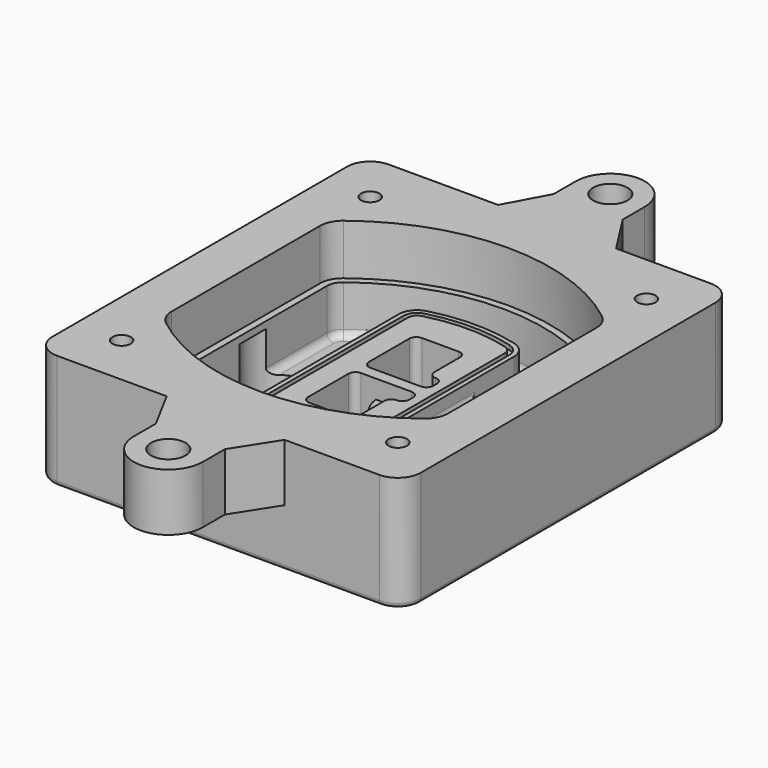
from build123d import *

# Parameters (mm, degrees)
F0_R      = 4
F1_DEPTH  = 25
F2_DEPTH  = 3
F3_DEPTH  = 18
F5_DEPTH  = 21
F6_DEPTH  = 2
F8_DEPTH  = 20
F9_DEPTH  = 16
F10_DEPTH = 25
F7_R      = 6
F7_R_2    = 4
F11_DEPTH = 6
F13_DEPTH = 9
F14_R     = 3
F15_R     = 2
F16_R     = 4
F17_DEPTH = 25
F18_DEPTH = 25
F19_DEPTH = 25
F16_R_2   = 7.5
F20_DEPTH = 25


# Not quite as in the source:
# - a feature names something its author has since deleted; it is built from what else it names


with BuildPart() as f1:
    # F0 (on Top) → F1 (new body)
    with BuildSketch(Plane.XY):
        with BuildLine():
            ThreePointArc((-80, -80), (-77.0710678119, -87.0710678119), (-70, -90))
            Line((-70, -90), (70, -90))
            ThreePointArc((70, -90), (77.0710678119, -87.0710678119), (80, -80))
            Line((80, -80), (80, 80))
            ThreePointArc((80, 80), (77.0710678119, 87.0710678119), (70, 90))
            Line((70, 90), (-70, 90))
            ThreePointArc((-70, 90), (-77.0710678119, 87.0710678119), (-80, 80))
            Line((-80, 80), (-80, -80))
        make_face()
        with Locations((-60, -67.5)):
            Circle(F0_R, mode=Mode.SUBTRACT)
        with Locations((60, -67.5)):
            Circle(F0_R, mode=Mode.SUBTRACT)
        with Locations((-60, 67.5)):
            Circle(F0_R, mode=Mode.SUBTRACT)
        with BuildLine():
            ThreePointArc((-64, 40.2934422872), (-62.5820384798, 46.4328484224), (-58.6153846154, 51.3286200352))
            ThreePointArc((-58.6153846154, 51.3286200352), (0, 71.5), (58.6153846154, 51.3286200352))
            ThreePointArc((58.6153846154, 51.3286200352), (62.5820384798, 46.4328484224), (64, 40.2934422872))
            Line((64, 40.2934422872), (64, -40.2934422872))
            ThreePointArc((64, -40.2934422872), (62.5820384798, -46.4328484224), (58.6153846154, -51.3286200352))
            ThreePointArc((58.6153846154, -51.3286200352), (0, -71.5), (-58.6153846154, -51.3286200352))
            ThreePointArc((-58.6153846154, -51.3286200352), (-62.5820384798, -46.4328484224), (-64, -40.2934422872))
            Line((-64, -40.2934422872), (-64, 40.2934422872))
        make_face(mode=Mode.SUBTRACT)
        with Locations((60, 67.5)):
            Circle(F0_R, mode=Mode.SUBTRACT)
        with BuildLine():
            ThreePointArc((58.6153846154, 51.3286200352), (0, 71.5), (-58.6153846154, 51.3286200352))
            ThreePointArc((-58.6153846154, 51.3286200352), (-62.5820384798, 46.4328484224), (-64, 40.2934422872))
            Line((-64, 40.2934422872), (-64, -40.2934422872))
            ThreePointArc((-64, -40.2934422872), (-62.5820384798, -46.4328484224), (-58.6153846154, -51.3286200352))
            ThreePointArc((-58.6153846154, -51.3286200352), (0, -71.5), (58.6153846154, -51.3286200352))
            ThreePointArc((58.6153846154, -51.3286200352), (62.5820384798, -46.4328484224), (64, -40.2934422872))
            Line((64, -40.2934422872), (64, 40.2934422872))
            ThreePointArc((64, 40.2934422872), (62.5820384798, 46.4328484224), (58.6153846154, 51.3286200352))
        make_face()
        with BuildLine():
            Line((-60, -40.2934422872), (-60, 40.2934422872))
            ThreePointArc((-60, 40.2934422872), (-58.9871703427, 44.6787323838), (-56.1538461538, 48.1757121072))
            ThreePointArc((-56.1538461538, 48.1757121072), (0, 67.5), (56.1538461538, 48.1757121072))
            ThreePointArc((56.1538461538, 48.1757121072), (58.9871703427, 44.6787323838), (60, 40.2934422872))
            Line((60, 40.2934422872), (60, -40.2934422872))
            ThreePointArc((60, -40.2934422872), (58.9871703427, -44.6787323838), (56.1538461538, -48.1757121072))
            ThreePointArc((56.1538461538, -48.1757121072), (0, -67.5), (-56.1538461538, -48.1757121072))
            ThreePointArc((-56.1538461538, -48.1757121072), (-58.9871703427, -44.6787323838), (-60, -40.2934422872))
        make_face(mode=Mode.SUBTRACT)
        with BuildLine():
            ThreePointArc((-56.1538461538, 48.1757121072), (-58.9871703427, 44.6787323838), (-60, 40.2934422872))
            Line((-60, 40.2934422872), (-60, -40.2934422872))
            ThreePointArc((-60, -40.2934422872), (-58.9871703427, -44.6787323838), (-56.1538461538, -48.1757121072))
            ThreePointArc((-56.1538461538, -48.1757121072), (0, -67.5), (56.1538461538, -48.1757121072))
            ThreePointArc((56.1538461538, -48.1757121072), (58.9871703427, -44.6787323838), (60, -40.2934422872))
            Line((60, -40.2934422872), (60, 40.2934422872))
            ThreePointArc((60, 40.2934422872), (58.9871703427, 44.6787323838), (56.1538461538, 48.1757121072))
            ThreePointArc((56.1538461538, 48.1757121072), (0, 67.5), (-56.1538461538, 48.1757121072))
        make_face()
        with BuildLine():
            ThreePointArc((54.3076923077, 45.8110311612), (56.2910192399, 43.3631453548), (57, 40.2934422872))
            Line((57, 40.2934422872), (57, -40.2934422872))
            ThreePointArc((57, -40.2934422872), (56.2910192399, -43.3631453548), (54.3076923077, -45.8110311612))
            ThreePointArc((54.3076923077, -45.8110311612), (0, -64.5), (-54.3076923077, -45.8110311612))
            ThreePointArc((-54.3076923077, -45.8110311612), (-56.2910192399, -43.3631453548), (-57, -40.2934422872))
            Line((-57, -40.2934422872), (-57, 40.2934422872))
            ThreePointArc((-57, 40.2934422872), (-56.2910192399, 43.3631453548), (-54.3076923077, 45.8110311612))
            ThreePointArc((-54.3076923077, 45.8110311612), (0, 64.5), (54.3076923077, 45.8110311612))
        make_face(mode=Mode.SUBTRACT)
        with BuildLine():
            Line((57, -40.2934422872), (57, 40.2934422872))
            ThreePointArc((57, 40.2934422872), (56.2910192399, 43.3631453548), (54.3076923077, 45.8110311612))
            ThreePointArc((54.3076923077, 45.8110311612), (0, 64.5), (-54.3076923077, 45.8110311612))
            ThreePointArc((-54.3076923077, 45.8110311612), (-56.2910192399, 43.3631453548), (-57, 40.2934422872))
            Line((-57, 40.2934422872), (-57, -40.2934422872))
            ThreePointArc((-57, -40.2934422872), (-56.2910192399, -43.3631453548), (-54.3076923077, -45.8110311612))
            ThreePointArc((-54.3076923077, -45.8110311612), (0, -64.5), (54.3076923077, -45.8110311612))
            ThreePointArc((54.3076923077, -45.8110311612), (56.2910192399, -43.3631453548), (57, -40.2934422872))
        make_face()
    extrude(amount=-F1_DEPTH)

    # F0 (on Top) → F2 (join)
    with BuildSketch(Plane.XY):
        with BuildLine():
            ThreePointArc((-56.1538461538, 48.1757121072), (-58.9871703427, 44.6787323838), (-60, 40.2934422872))
            Line((-60, 40.2934422872), (-60, -40.2934422872))
            ThreePointArc((-60, -40.2934422872), (-58.9871703427, -44.6787323838), (-56.1538461538, -48.1757121072))
            ThreePointArc((-56.1538461538, -48.1757121072), (0, -67.5), (56.1538461538, -48.1757121072))
            ThreePointArc((56.1538461538, -48.1757121072), (58.9871703427, -44.6787323838), (60, -40.2934422872))
            Line((60, -40.2934422872), (60, 40.2934422872))
            ThreePointArc((60, 40.2934422872), (58.9871703427, 44.6787323838), (56.1538461538, 48.1757121072))
            ThreePointArc((56.1538461538, 48.1757121072), (0, 67.5), (-56.1538461538, 48.1757121072))
        make_face()
        with BuildLine():
            ThreePointArc((54.3076923077, 45.8110311612), (56.2910192399, 43.3631453548), (57, 40.2934422872))
            Line((57, 40.2934422872), (57, -40.2934422872))
            ThreePointArc((57, -40.2934422872), (56.2910192399, -43.3631453548), (54.3076923077, -45.8110311612))
            ThreePointArc((54.3076923077, -45.8110311612), (0, -64.5), (-54.3076923077, -45.8110311612))
            ThreePointArc((-54.3076923077, -45.8110311612), (-56.2910192399, -43.3631453548), (-57, -40.2934422872))
            Line((-57, -40.2934422872), (-57, 40.2934422872))
            ThreePointArc((-57, 40.2934422872), (-56.2910192399, 43.3631453548), (-54.3076923077, 45.8110311612))
            ThreePointArc((-54.3076923077, 45.8110311612), (0, 64.5), (54.3076923077, 45.8110311612))
        make_face(mode=Mode.SUBTRACT)
    extrude(amount=F2_DEPTH)

    # F0 (on Top) → F3 (cut)
    with BuildSketch(Plane.XY):
        with BuildLine():
            Line((57, -40.2934422872), (57, 40.2934422872))
            ThreePointArc((57, 40.2934422872), (56.2910192399, 43.3631453548), (54.3076923077, 45.8110311612))
            ThreePointArc((54.3076923077, 45.8110311612), (0, 64.5), (-54.3076923077, 45.8110311612))
            ThreePointArc((-54.3076923077, 45.8110311612), (-56.2910192399, 43.3631453548), (-57, 40.2934422872))
            Line((-57, 40.2934422872), (-57, -40.2934422872))
            ThreePointArc((-57, -40.2934422872), (-56.2910192399, -43.3631453548), (-54.3076923077, -45.8110311612))
            ThreePointArc((-54.3076923077, -45.8110311612), (0, -64.5), (54.3076923077, -45.8110311612))
            ThreePointArc((54.3076923077, -45.8110311612), (56.2910192399, -43.3631453548), (57, -40.2934422872))
        make_face()
    extrude(amount=-F3_DEPTH, mode=Mode.SUBTRACT)

    # F4 (on face) → F5 (join, through all)
    with BuildSketch(Plane.XY.offset(3)):
        with BuildLine():
            ThreePointArc((-25, -39.2465276821), (-23.3511545998, -44.1109737193), (-19.0842911877, -46.9702398883))
            ThreePointArc((-19.0842911877, -46.9702398883), (0, -49.5), (19.0842911877, -46.9702398883))
            ThreePointArc((19.0842911877, -46.9702398883), (23.3511545998, -44.1109737193), (25, -39.2465276821))
            Line((25, -39.2465276821), (25, 39.2465276821))
            ThreePointArc((25, 39.2465276821), (23.3511545998, 44.1109737193), (19.0842911877, 46.9702398883))
            ThreePointArc((19.0842911877, 46.9702398883), (0, 49.5), (-19.0842911877, 46.9702398883))
            ThreePointArc((-19.0842911877, 46.9702398883), (-23.3511545998, 44.1109737193), (-25, 39.2465276821))
            Line((-25, 39.2465276821), (-25, -39.2465276821))
        make_face()
        with BuildLine():
            ThreePointArc((18.5632183908, 45.0393118368), (21.7633659499, 42.89486221), (23, 39.2465276821))
            Line((23, 39.2465276821), (23, -39.2465276821))
            ThreePointArc((23, -39.2465276821), (21.7633659499, -42.89486221), (18.5632183908, -45.0393118368))
            ThreePointArc((18.5632183908, -45.0393118368), (0, -47.5), (-18.5632183908, -45.0393118368))
            ThreePointArc((-18.5632183908, -45.0393118368), (-21.7633659499, -42.89486221), (-23, -39.2465276821))
            Line((-23, -39.2465276821), (-23, 39.2465276821))
            ThreePointArc((-23, 39.2465276821), (-21.7633659499, 42.89486221), (-18.5632183908, 45.0393118368))
            ThreePointArc((-18.5632183908, 45.0393118368), (0, 47.5), (18.5632183908, 45.0393118368))
        make_face(mode=Mode.SUBTRACT)
        with BuildLine():
            Line((23, -39.2465276821), (23, 39.2465276821))
            ThreePointArc((23, 39.2465276821), (21.7633659499, 42.89486221), (18.5632183908, 45.0393118368))
            ThreePointArc((18.5632183908, 45.0393118368), (0, 47.5), (-18.5632183908, 45.0393118368))
            ThreePointArc((-18.5632183908, 45.0393118368), (-21.7633659499, 42.89486221), (-23, 39.2465276821))
            Line((-23, 39.2465276821), (-23, -39.2465276821))
            ThreePointArc((-23, -39.2465276821), (-21.7633659499, -42.89486221), (-18.5632183908, -45.0393118368))
            ThreePointArc((-18.5632183908, -45.0393118368), (0, -47.5), (18.5632183908, -45.0393118368))
            ThreePointArc((18.5632183908, -45.0393118368), (21.7633659499, -42.89486221), (23, -39.2465276821))
        make_face()
        with BuildLine():
            ThreePointArc((18.0421455939, 43.1083837852), (20.1755772999, 41.6787507007), (21, 39.2465276821))
            Line((21, 39.2465276821), (21, -39.2465276821))
            ThreePointArc((21, -39.2465276821), (20.1755772999, -41.6787507007), (18.0421455939, -43.1083837852))
            ThreePointArc((18.0421455939, -43.1083837852), (0, -45.5), (-18.0421455939, -43.1083837852))
            ThreePointArc((-18.0421455939, -43.1083837852), (-20.1755772999, -41.6787507007), (-21, -39.2465276821))
            Line((-21, -39.2465276821), (-21, 39.2465276821))
            ThreePointArc((-21, 39.2465276821), (-20.1755772999, 41.6787507007), (-18.0421455939, 43.1083837852))
            ThreePointArc((-18.0421455939, 43.1083837852), (0, 45.5), (18.0421455939, 43.1083837852))
        make_face(mode=Mode.SUBTRACT)
        with BuildLine():
            Line((21, -39.2465276821), (21, 39.2465276821))
            ThreePointArc((21, 39.2465276821), (20.1755772999, 41.6787507007), (18.0421455939, 43.1083837852))
            ThreePointArc((18.0421455939, 43.1083837852), (0, 45.5), (-18.0421455939, 43.1083837852))
            ThreePointArc((-18.0421455939, 43.1083837852), (-20.1755772999, 41.6787507007), (-21, 39.2465276821))
            Line((-21, 39.2465276821), (-21, -39.2465276821))
            ThreePointArc((-21, -39.2465276821), (-20.1755772999, -41.6787507007), (-18.0421455939, -43.1083837852))
            ThreePointArc((-18.0421455939, -43.1083837852), (0, -45.5), (18.0421455939, -43.1083837852))
            ThreePointArc((18.0421455939, -43.1083837852), (20.1755772999, -41.6787507007), (21, -39.2465276821))
        make_face()
        with BuildLine():
            Line((-8, -2.5), (14, -2.5))
            ThreePointArc((14, -2.5), (16.1213203436, -3.3786796564), (17, -5.5))
            Line((17, -5.5), (17, -7.5))
            ThreePointArc((17, -7.5), (16.1213203436, -9.6213203436), (14, -10.5))
            ThreePointArc((14, -10.5), (11.8786796564, -11.3786796564), (11, -13.5))
            Line((11, -13.5), (11, -27.5))
            ThreePointArc((11, -27.5), (10.1213203436, -29.6213203436), (8, -30.5))
            Line((8, -30.5), (-8, -30.5))
            ThreePointArc((-8, -30.5), (-10.1213203436, -29.6213203436), (-11, -27.5))
            Line((-11, -27.5), (-11, -5.5))
            ThreePointArc((-11, -5.5), (-10.1213203436, -3.3786796564), (-8, -2.5))
        make_face(mode=Mode.SUBTRACT)
        with BuildLine():
            ThreePointArc((-8, 2.5), (-10.1213203436, 3.3786796564), (-11, 5.5))
            Line((-11, 5.5), (-11, 27.5))
            ThreePointArc((-11, 27.5), (-10.1213203436, 29.6213203436), (-8, 30.5))
            Line((-8, 30.5), (8, 30.5))
            ThreePointArc((8, 30.5), (10.1213203436, 29.6213203436), (11, 27.5))
            Line((11, 27.5), (11, 13.5))
            ThreePointArc((11, 13.5), (11.8786796564, 11.3786796564), (14, 10.5))
            ThreePointArc((14, 10.5), (16.1213203436, 9.6213203436), (17, 7.5))
            Line((17, 7.5), (17, 5.5))
            ThreePointArc((17, 5.5), (16.1213203436, 3.3786796564), (14, 2.5))
            Line((14, 2.5), (-8, 2.5))
        make_face(mode=Mode.SUBTRACT)
    extrude(amount=-F5_DEPTH)

    # F4 (on face) → F6 (cut)
    with BuildSketch(Plane.XY.offset(3)):
        with BuildLine():
            Line((23, -39.2465276821), (23, 39.2465276821))
            ThreePointArc((23, 39.2465276821), (21.7633659499, 42.89486221), (18.5632183908, 45.0393118368))
            ThreePointArc((18.5632183908, 45.0393118368), (0, 47.5), (-18.5632183908, 45.0393118368))
            ThreePointArc((-18.5632183908, 45.0393118368), (-21.7633659499, 42.89486221), (-23, 39.2465276821))
            Line((-23, 39.2465276821), (-23, -39.2465276821))
            ThreePointArc((-23, -39.2465276821), (-21.7633659499, -42.89486221), (-18.5632183908, -45.0393118368))
            ThreePointArc((-18.5632183908, -45.0393118368), (0, -47.5), (18.5632183908, -45.0393118368))
            ThreePointArc((18.5632183908, -45.0393118368), (21.7633659499, -42.89486221), (23, -39.2465276821))
        make_face()
        with BuildLine():
            ThreePointArc((18.0421455939, 43.1083837852), (20.1755772999, 41.6787507007), (21, 39.2465276821))
            Line((21, 39.2465276821), (21, -39.2465276821))
            ThreePointArc((21, -39.2465276821), (20.1755772999, -41.6787507007), (18.0421455939, -43.1083837852))
            ThreePointArc((18.0421455939, -43.1083837852), (0, -45.5), (-18.0421455939, -43.1083837852))
            ThreePointArc((-18.0421455939, -43.1083837852), (-20.1755772999, -41.6787507007), (-21, -39.2465276821))
            Line((-21, -39.2465276821), (-21, 39.2465276821))
            ThreePointArc((-21, 39.2465276821), (-20.1755772999, 41.6787507007), (-18.0421455939, 43.1083837852))
            ThreePointArc((-18.0421455939, 43.1083837852), (0, 45.5), (18.0421455939, 43.1083837852))
        make_face(mode=Mode.SUBTRACT)
    extrude(amount=-F6_DEPTH, mode=Mode.SUBTRACT)

    # F7 (on face) → F8 (join)
    with BuildSketch(Plane(origin=(0, 0, -25), x_dir=(1, 0, 0), z_dir=(0, 0, -1))):
        with BuildLine():
            ThreePointArc((3.28842436, 0), (16.7567035675, 13.4682792075), (30.224982775, 0))
            Line((30.224982775, 0), (35.224982775, 0))
            ThreePointArc((35.224982775, 0), (16.7567035675, 18.4682792075), (-1.71157564, 0))
            Line((-1.71157564, 0), (3.28842436, 0))
        make_face()
        with BuildLine():
            Line((3.28842436, 0), (30.224982775, 0))
            ThreePointArc((30.224982775, 0), (16.7567035675, 13.4682792075), (3.28842436, 0))
        make_face()
        with BuildLine():
            ThreePointArc((3.28842436, 0), (16.7567035675, -13.4682792075), (30.224982775, 0))
            Line((30.224982775, 0), (3.28842436, 0))
        make_face()
        with BuildLine():
            Line((35.224982775, 0), (30.224982775, 0))
            ThreePointArc((30.224982775, 0), (16.7567035675, -13.4682792075), (3.28842436, 0))
            Line((3.28842436, 0), (-1.71157564, 0))
            ThreePointArc((-1.71157564, 0), (16.7567035675, -18.4682792075), (35.224982775, 0))
        make_face()
    extrude(amount=-F8_DEPTH)

    # F7 (on face) → F9 (cut)
    with BuildSketch(Plane(origin=(0, 0, -25), x_dir=(1, 0, 0), z_dir=(0, 0, -1))):
        with BuildLine():
            Line((3.28842436, 0), (30.224982775, 0))
            ThreePointArc((30.224982775, 0), (16.7567035675, 13.4682792075), (3.28842436, 0))
        make_face()
        with BuildLine():
            ThreePointArc((3.28842436, 0), (16.7567035675, -13.4682792075), (30.224982775, 0))
            Line((30.224982775, 0), (3.28842436, 0))
        make_face()
    extrude(amount=-F9_DEPTH, mode=Mode.SUBTRACT)

    # F7 (on face) → F10 (cut)
    with BuildSketch(Plane(origin=(0, 0, -25), x_dir=(1, 0, 0), z_dir=(0, 0, -1))):
        with BuildLine():
            Line((-59.0318229325, 0), (-32.0952645175, 0))
            ThreePointArc((-32.0952645175, 0), (-45.563543725, 13.4682792075), (-59.0318229325, 0))
        make_face()
        with BuildLine():
            ThreePointArc((-59.0318229325, 0), (-45.563543725, -13.4682792075), (-32.0952645175, 0))
            Line((-32.0952645175, 0), (-59.0318229325, 0))
        make_face()
    extrude(amount=-F10_DEPTH, mode=Mode.SUBTRACT)

    # F7 (on face) → F11 (cut)
    with BuildSketch(Plane(origin=(0, 0, -25), x_dir=(1, 0, 0), z_dir=(0, 0, -1))):
        with Locations((60, -67.5)):
            Circle(F7_R)
        with Locations((60, -67.5)):
            Circle(F7_R_2, mode=Mode.SUBTRACT)
        with Locations((-60, -67.5)):
            Circle(F7_R)
        with Locations((-60, -67.5)):
            Circle(F7_R_2, mode=Mode.SUBTRACT)
        with Locations((-60, 67.5)):
            Circle(F7_R)
        with Locations((-60, 67.5)):
            Circle(F7_R_2, mode=Mode.SUBTRACT)
        with Locations((60, 67.5)):
            Circle(F7_R)
        with Locations((60, 67.5)):
            Circle(F7_R_2, mode=Mode.SUBTRACT)
    extrude(amount=-F11_DEPTH, mode=Mode.SUBTRACT)

    # F12 (on face) → F13 (cut, through all)
    with BuildSketch(Plane(origin=(0, 0, -9), x_dir=(1, 0, 0), z_dir=(0, 0, -1))):
        with BuildLine():
            Line((11, 13.5), (11, 17.5481537753))
            ThreePointArc((11, 17.5481537753), (2.5696536419, 11.8239143813), (-1.5415842455, 2.5))
            Line((-1.5415842455, 2.5), (3.5224848595, 2.5))
            ThreePointArc((3.5224848595, 2.5), (6.1857188154, 8.3455872281), (11.2536447004, 12.2927168648))
            ThreePointArc((11.2536447004, 12.2927168648), (11.0640958889, 12.8831798879), (11, 13.5))
        make_face()
        with BuildLine():
            ThreePointArc((11.2536447004, -12.2927168648), (6.1857188154, -8.3455872281), (3.5224848595, -2.5))
            Line((3.5224848595, -2.5), (-1.5415842455, -2.5))
            ThreePointArc((-1.5415842455, -2.5), (2.5696536419, -11.8239143813), (11, -17.5481537753))
            Line((11, -17.5481537753), (11, -13.5))
            ThreePointArc((11, -13.5), (11.0640958889, -12.8831798879), (11.2536447004, -12.2927168648))
        make_face()
        with BuildLine():
            ThreePointArc((11.2536447004, 12.2927168648), (6.1857188154, 8.3455872281), (3.5224848595, 2.5))
            Line((3.5224848595, 2.5), (14, 2.5))
            ThreePointArc((14, 2.5), (16.1213203436, 3.3786796564), (17, 5.5))
            Line((17, 5.5), (17, 7.5))
            ThreePointArc((17, 7.5), (16.1213203436, 9.6213203436), (14, 10.5))
            ThreePointArc((14, 10.5), (12.3601599782, 10.9878446101), (11.2536447004, 12.2927168648))
        make_face()
        with BuildLine():
            Line((14, -2.5), (3.5224848595, -2.5))
            ThreePointArc((3.5224848595, -2.5), (6.1857188154, -8.3455872281), (11.2536447004, -12.2927168648))
            ThreePointArc((11.2536447004, -12.2927168648), (12.3601599782, -10.9878446101), (14, -10.5))
            ThreePointArc((14, -10.5), (16.1213203436, -9.6213203436), (17, -7.5))
            Line((17, -7.5), (17, -5.5))
            ThreePointArc((17, -5.5), (16.1213203436, -3.3786796564), (14, -2.5))
        make_face()
    extrude(amount=F13_DEPTH, mode=Mode.SUBTRACT)

    # F14
    f14_edges = [f1.edges().sort_by_distance(p)[0] for p in [
        (-57, -23.703476, -18),
        (-57, 23.703476, -18),
        (25, 0, -5),
        (25, 16.526506, -11.5),
        (25, -16.526506, -11.5),
        (25, -27.886517, -18),
        (35.224983, 0, -18),
    ]]
    fillet(f14_edges, radius=F14_R)

    # F15
    f15_edges = [f1.edges().sort_by_distance(p)[0] for p in [
        (0, -90, -25),
    ]]
    fillet(f15_edges, radius=F15_R)

    # F16 (on face) → F17 (join)
    with BuildSketch(Plane.XY):
        with BuildLine():
            Line((28.8198757917, 90), (-22.4184465061, 90))
            Line((-22.4184465061, 90), (-70, 90))
            ThreePointArc((-70, 90), (-77.0710678119, 87.0710678119), (-80, 80))
            Line((-80, 80), (-80, -80))
            ThreePointArc((-80, -80), (-77.0710678119, -87.0710678119), (-70, -90))
            Line((-70, -90), (-22.4184465061, -90))
            Line((-22.4184465061, -90), (28.8198757917, -90))
            Line((28.8198757917, -90), (70, -90))
            ThreePointArc((70, -90), (77.0710678119, -87.0710678119), (80, -80))
            Line((80, -80), (80, 80))
            ThreePointArc((80, 80), (77.0710678119, 87.0710678119), (70, 90))
            Line((70, 90), (28.8198757917, 90))
        make_face()
        with Locations((-60, -67.5)):
            Circle(F16_R, mode=Mode.SUBTRACT)
        with Locations((60, -67.5)):
            Circle(F16_R, mode=Mode.SUBTRACT)
        with Locations((-60, 67.5)):
            Circle(F16_R, mode=Mode.SUBTRACT)
        with BuildLine():
            ThreePointArc((-60, 40.2934422872), (-58.9871703427, 44.6787323838), (-56.1538461538, 48.1757121072))
            ThreePointArc((-56.1538461538, 48.1757121072), (0, 67.5), (56.1538461538, 48.1757121072))
            ThreePointArc((56.1538461538, 48.1757121072), (58.9871703427, 44.6787323838), (60, 40.2934422872))
            Line((60, 40.2934422872), (60, -40.2934422872))
            ThreePointArc((60, -40.2934422872), (58.9871703427, -44.6787323838), (56.1538461538, -48.1757121072))
            ThreePointArc((56.1538461538, -48.1757121072), (0, -67.5), (-56.1538461538, -48.1757121072))
            ThreePointArc((-56.1538461538, -48.1757121072), (-58.9871703427, -44.6787323838), (-60, -40.2934422872))
            Line((-60, -40.2934422872), (-60, 40.2934422872))
        make_face(mode=Mode.SUBTRACT)
        with Locations((60, 67.5)):
            Circle(F16_R, mode=Mode.SUBTRACT)
    extrude(amount=F17_DEPTH)

    # F16 (on face) → F18 (join)
    with BuildSketch(Plane.XY):
        with BuildLine():
            Line((28.8198757917, 90), (-22.4184465061, 90))
            Line((-22.4184465061, 90), (-70, 90))
            ThreePointArc((-70, 90), (-77.0710678119, 87.0710678119), (-80, 80))
            Line((-80, 80), (-80, -80))
            ThreePointArc((-80, -80), (-77.0710678119, -87.0710678119), (-70, -90))
            Line((-70, -90), (-22.4184465061, -90))
            Line((-22.4184465061, -90), (28.8198757917, -90))
            Line((28.8198757917, -90), (70, -90))
            ThreePointArc((70, -90), (77.0710678119, -87.0710678119), (80, -80))
            Line((80, -80), (80, 80))
            ThreePointArc((80, 80), (77.0710678119, 87.0710678119), (70, 90))
            Line((70, 90), (28.8198757917, 90))
        make_face()
        with Locations((-60, -67.5)):
            Circle(F16_R, mode=Mode.SUBTRACT)
        with Locations((60, -67.5)):
            Circle(F16_R, mode=Mode.SUBTRACT)
        with Locations((-60, 67.5)):
            Circle(F16_R, mode=Mode.SUBTRACT)
        with BuildLine():
            ThreePointArc((-60, 40.2934422872), (-58.9871703427, 44.6787323838), (-56.1538461538, 48.1757121072))
            ThreePointArc((-56.1538461538, 48.1757121072), (0, 67.5), (56.1538461538, 48.1757121072))
            ThreePointArc((56.1538461538, 48.1757121072), (58.9871703427, 44.6787323838), (60, 40.2934422872))
            Line((60, 40.2934422872), (60, -40.2934422872))
            ThreePointArc((60, -40.2934422872), (58.9871703427, -44.6787323838), (56.1538461538, -48.1757121072))
            ThreePointArc((56.1538461538, -48.1757121072), (0, -67.5), (-56.1538461538, -48.1757121072))
            ThreePointArc((-56.1538461538, -48.1757121072), (-58.9871703427, -44.6787323838), (-60, -40.2934422872))
            Line((-60, -40.2934422872), (-60, 40.2934422872))
        make_face(mode=Mode.SUBTRACT)
        with Locations((60, 67.5)):
            Circle(F16_R, mode=Mode.SUBTRACT)
    extrude(amount=F18_DEPTH)

    # F16 (on face) → F19 (join)
    with BuildSketch(Plane.XY):
        with BuildLine():
            Line((28.8198757917, 90), (-22.4184465061, 90))
            Line((-22.4184465061, 90), (-70, 90))
            ThreePointArc((-70, 90), (-77.0710678119, 87.0710678119), (-80, 80))
            Line((-80, 80), (-80, -80))
            ThreePointArc((-80, -80), (-77.0710678119, -87.0710678119), (-70, -90))
            Line((-70, -90), (-22.4184465061, -90))
            Line((-22.4184465061, -90), (28.8198757917, -90))
            Line((28.8198757917, -90), (70, -90))
            ThreePointArc((70, -90), (77.0710678119, -87.0710678119), (80, -80))
            Line((80, -80), (80, 80))
            ThreePointArc((80, 80), (77.0710678119, 87.0710678119), (70, 90))
            Line((70, 90), (28.8198757917, 90))
        make_face()
        with Locations((-60, -67.5)):
            Circle(F16_R, mode=Mode.SUBTRACT)
        with Locations((60, -67.5)):
            Circle(F16_R, mode=Mode.SUBTRACT)
        with Locations((-60, 67.5)):
            Circle(F16_R, mode=Mode.SUBTRACT)
        with BuildLine():
            ThreePointArc((-60, 40.2934422872), (-58.9871703427, 44.6787323838), (-56.1538461538, 48.1757121072))
            ThreePointArc((-56.1538461538, 48.1757121072), (0, 67.5), (56.1538461538, 48.1757121072))
            ThreePointArc((56.1538461538, 48.1757121072), (58.9871703427, 44.6787323838), (60, 40.2934422872))
            Line((60, 40.2934422872), (60, -40.2934422872))
            ThreePointArc((60, -40.2934422872), (58.9871703427, -44.6787323838), (56.1538461538, -48.1757121072))
            ThreePointArc((56.1538461538, -48.1757121072), (0, -67.5), (-56.1538461538, -48.1757121072))
            ThreePointArc((-56.1538461538, -48.1757121072), (-58.9871703427, -44.6787323838), (-60, -40.2934422872))
            Line((-60, -40.2934422872), (-60, 40.2934422872))
        make_face(mode=Mode.SUBTRACT)
        with Locations((60, 67.5)):
            Circle(F16_R, mode=Mode.SUBTRACT)
    extrude(amount=F19_DEPTH)

    # F16 (on face) → F20 (join)
    with BuildSketch(Plane.XY):
        with BuildLine():
            Line((28.8198757917, 90), (-22.4184465061, 90))
            Line((-22.4184465061, 90), (-70, 90))
            ThreePointArc((-70, 90), (-77.0710678119, 87.0710678119), (-80, 80))
            Line((-80, 80), (-80, -80))
            ThreePointArc((-80, -80), (-77.0710678119, -87.0710678119), (-70, -90))
            Line((-70, -90), (-22.4184465061, -90))
            Line((-22.4184465061, -90), (28.8198757917, -90))
            Line((28.8198757917, -90), (70, -90))
            ThreePointArc((70, -90), (77.0710678119, -87.0710678119), (80, -80))
            Line((80, -80), (80, 80))
            ThreePointArc((80, 80), (77.0710678119, 87.0710678119), (70, 90))
            Line((70, 90), (28.8198757917, 90))
        make_face()
        with Locations((-60, -67.5)):
            Circle(F16_R, mode=Mode.SUBTRACT)
        with Locations((60, -67.5)):
            Circle(F16_R, mode=Mode.SUBTRACT)
        with Locations((-60, 67.5)):
            Circle(F16_R, mode=Mode.SUBTRACT)
        with BuildLine():
            ThreePointArc((-60, 40.2934422872), (-58.9871703427, 44.6787323838), (-56.1538461538, 48.1757121072))
            ThreePointArc((-56.1538461538, 48.1757121072), (0, 67.5), (56.1538461538, 48.1757121072))
            ThreePointArc((56.1538461538, 48.1757121072), (58.9871703427, 44.6787323838), (60, 40.2934422872))
            Line((60, 40.2934422872), (60, -40.2934422872))
            ThreePointArc((60, -40.2934422872), (58.9871703427, -44.6787323838), (56.1538461538, -48.1757121072))
            ThreePointArc((56.1538461538, -48.1757121072), (0, -67.5), (-56.1538461538, -48.1757121072))
            ThreePointArc((-56.1538461538, -48.1757121072), (-58.9871703427, -44.6787323838), (-60, -40.2934422872))
            Line((-60, -40.2934422872), (-60, 40.2934422872))
        make_face(mode=Mode.SUBTRACT)
        with Locations((60, 67.5)):
            Circle(F16_R, mode=Mode.SUBTRACT)
        with BuildLine():
            Line((28.8198757917, -90), (-22.4184465061, -90))
            Line((-22.4184465061, -90), (-12.7026606351, -108))
            Line((-12.7026606351, -108), (-12.7026606351, -120))
            ThreePointArc((-12.7026606351, -120), (2.3164321868, -134.9999878488), (17.2972907601, -119.9618143871))
            Line((17.2972907601, -119.9618143871), (17.2972907601, -108))
            Line((17.2972907601, -108), (28.8198757917, -90))
        make_face()
        with Locations((2.2973393649, -120)):
            Circle(F16_R_2, mode=Mode.SUBTRACT)
        with BuildLine():
            Line((-12.7026606351, 108), (-22.4184465061, 90))
            Line((-22.4184465061, 90), (28.8198757917, 90))
            Line((28.8198757917, 90), (17.2972907601, 108))
            Line((17.2972907601, 108), (17.2972907601, 119.9618143871))
            ThreePointArc((17.2972907601, 119.9618143871), (2.3164321868, 134.9999878488), (-12.7026606351, 120))
            Line((-12.7026606351, 120), (-12.7026606351, 108))
        make_face()
        with Locations((2.2973393649, 120)):
            Circle(F16_R_2, mode=Mode.SUBTRACT)
    extrude(amount=F20_DEPTH)


solid = f1.part
